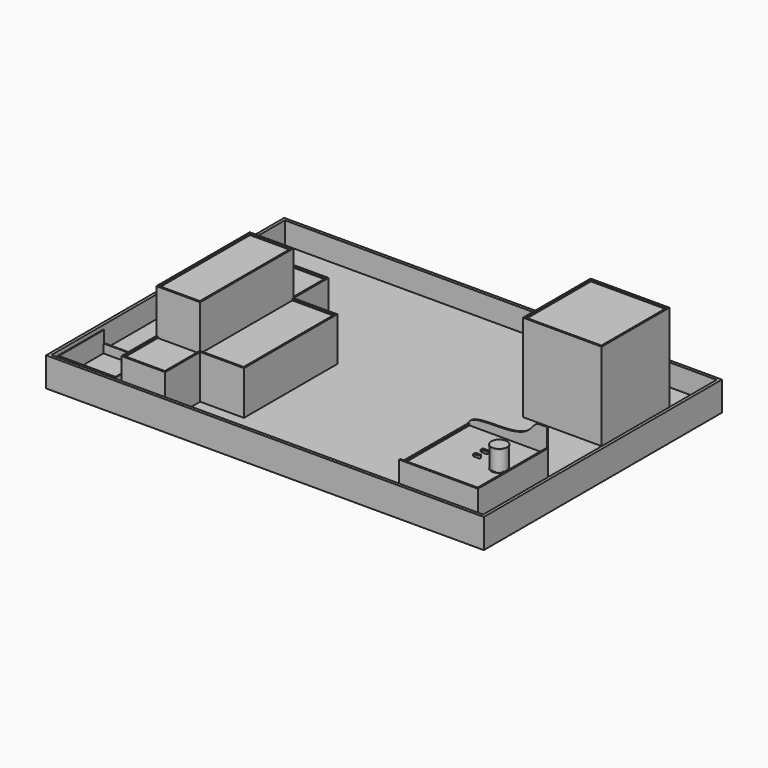
from build123d import *

# Parameters (mm, degrees)
F0_R      = 27.2
F1_DEPTH  = 2.83
F2_R      = 26.4
F3_DEPTH  = 67.36
F4_R      = 27.2
F5_DEPTH  = 2.83
F9_W      = 270
F9_H      = 300
F10_DEPTH = 72
F12_DEPTH = 15
F14_DEPTH = 5
F15_W     = 5
F15_H     = 290
F16_DEPTH = 5
F17_W     = 1500
F17_H     = 1020
F18_DEPTH = 25
F19_W     = 270
F19_H     = 290
F20_DEPTH = 300
F21_W     = 260
F21_H     = 280
F22_DEPTH = 5
F23_W     = 1500
F23_H     = 1020
F23_W_2   = 1480
F23_H_2   = 1000
F24_DEPTH = 75
F26_DEPTH = 150
F27_W     = 150
F27_H     = 400
F28_DEPTH = 150
F29_W     = 140
F29_H     = 390
F30_DEPTH = 5
F31_W     = 140
F31_H     = 145
F31_W_2   = 145
F31_H_2   = 390
F32_DEPTH = 5
F33_R     = 3
F34_DEPTH = 4
F35_R     = 3.99999
F35_2_R   = 3.99999
F36_R     = 3
F37_DEPTH = 8
F38_R     = 3
F39_DEPTH = 8
F40_R     = 3
F40_R_2   = 2.5
F41_DEPTH = 3
F42_R     = 3
F42_R_2   = 2.5
F43_DEPTH = 3
F45_DEPTH = 270.001
F46_W     = 200
F46_H     = 200
F46_W_2   = 194
F46_H_2   = 191
F47_DEPTH = 30
F49_DEPTH = 40
F50_R     = 2.5
F51_DEPTH = 8


# Not quite as in the source:
# - a fillet or chamfer is up to 0.001 mm smaller than in the source, because OpenCascade refuses the exact size
# - a feature names something its author has since deleted; it is built from what else it names


with BuildPart() as f1:
    # F0 (on Top) → F1 (new body)
    with BuildSketch(Plane.XY):
        Circle(F0_R)
    extrude(amount=F1_DEPTH)

    # F2 (on face) → F3 (join)
    with BuildSketch(Plane.XY.offset(2.83)):
        Circle(F2_R)
    extrude(amount=F3_DEPTH)

    # F4 (on face) → F5 (join)
    with BuildSketch(Plane.XY.offset(70.19)):
        Circle(F4_R)
    extrude(amount=F5_DEPTH)


with BuildPart() as f10:
    # F9 (on Top) → F10 (new body)
    with BuildSketch(Plane.XY):
        with Locations((-87.8, 0)):
            Rectangle(F9_W, F9_H)
    extrude(amount=-F10_DEPTH)

    # F11 (on face) → F12 (join)
    with BuildSketch(Plane.XY):
        Polygon((-222.8, -145), (-222.8, -150), (47.2, -150), (47.2, 150), (42.2, 150), (42.2, -145), align=None)
    extrude(amount=F12_DEPTH)

    # F13 (on face) → F14 (join)
    with BuildSketch(Plane(origin=(0, 150, 0), x_dir=(-1, 0, 0), z_dir=(0, 1, 0))):
        with BuildLine():
            Line((-21.3134280931, 81.3575685024), (-47.2, 81.3575685024))
            Line((-47.2, 81.3575685024), (-47.2, -72))
            Line((-47.2, -72), (222.8, -72))
            Line((222.8, -72), (222.8, 0))
            add(Edge.make_bspline(
                [(-21.3134280931, 81.3575685024), (-6.3059147253, 81.3822787863), (12.9585432644, 38.1268753575), (103.6097013063, 23.6068887567), (223.0224295336, 30.7718731823), (222.8, 0)],
                knots=[0, 0, 0, 0, 0.2487100673, 0.6151112321, 1, 1, 1, 1], degree=3))
        make_face()
    extrude(amount=-F14_DEPTH)

    # F15 (on face) → F16 (join)
    with BuildSketch(Plane.XY):
        with Locations((-220.3, 0)):
            Rectangle(F15_W, F15_H)
    extrude(amount=F16_DEPTH)

    # F17 (on face) → F18 (join)
    with BuildSketch(Plane(origin=(0, 0, -72), x_dir=(1, 0, 0), z_dir=(0, 0, -1))):
        with Locations((-602.8, -260)):
            Rectangle(F17_W, F17_H)
    extrude(amount=F18_DEPTH)

    # F19 (on face) → F20 (join)
    with BuildSketch(Plane.XY.offset(-72)):
        with Locations((-87.8, 525)):
            Rectangle(F19_W, F19_H)
    extrude(amount=F20_DEPTH)

    # F21 (on face) → F22 (cut)
    with BuildSketch(Plane.XY.offset(228)):
        with Locations((-87.8, 525)):
            Rectangle(F21_W, F21_H)
    extrude(amount=-F22_DEPTH, mode=Mode.SUBTRACT)

    # F23 (on face) → F24 (join)
    with BuildSketch(Plane.XY.offset(-72)):
        with Locations((-602.8, 260)):
            Rectangle(F23_W, F23_H)
        with Locations((-602.8, 260)):
            Rectangle(F23_W_2, F23_H_2, mode=Mode.SUBTRACT)
    extrude(amount=F24_DEPTH)

    # F25 (on face) → F26 (join)
    with BuildSketch(Plane.XY.offset(-72)):
        Polygon((-952.8, 460), (-1102.8, 460), (-1102.8, -240), (-952.8, -240), (-952.8, -90), (-802.8, -90), (-802.8, 310), (-952.8, 310), align=None)
    extrude(amount=F26_DEPTH)

    # F27 (on face) → F28 (join)
    with BuildSketch(Plane.XY.offset(78)):
        with Locations((-1027.8, 110)):
            Rectangle(F27_W, F27_H)
    extrude(amount=F28_DEPTH)

    # F29 (on face) → F30 (cut)
    with BuildSketch(Plane.XY.offset(228)):
        with Locations((-1027.8, 110)):
            Rectangle(F29_W, F29_H)
    extrude(amount=-F30_DEPTH, mode=Mode.SUBTRACT)

    # F31 (on face) → F32 (cut)
    with BuildSketch(Plane.XY.offset(78)):
        with Locations((-1027.8, 382.5)):
            Rectangle(F31_W, F31_H)
        with Locations((-880.3, 110)):
            Rectangle(F31_W_2, F31_H_2)
        with Locations((-1027.8, -162.5)):
            Rectangle(F31_W, F31_H)
    extrude(amount=-F32_DEPTH, mode=Mode.SUBTRACT)

    # F46 (on face) → F47 (join)
    with BuildSketch(Plane.XY.offset(-72)):
        with Locations((-1232.8, -130)):
            Rectangle(F46_W, F46_H)
        with Locations((-1232.8, -128.5)):
            Rectangle(F46_W_2, F46_H_2, mode=Mode.SUBTRACT)
    extrude(amount=F47_DEPTH)

    # F48 (on face) → F49 (join)
    with BuildSketch(Plane.XY.offset(-42)):
        Polygon((-1329.8, -30), (-1332.8, -30), (-1332.8, -230), (-1329.8, -230), (-1135.8, -230), (-1132.8, -230), (-1132.8, -30), (-1135.8, -30), (-1135.8, -224), (-1329.8, -224), align=None)
    extrude(amount=F49_DEPTH)


with BuildPart() as f34:
    # F33 (on offset) → F34 (new body, symmetric)
    with BuildSketch(Plane.XY.offset(25)):
        with BuildLine():
            Line((-55, -12), (-74.5, -12))
            Line((-74.5, -12), (-74.5, -13))
            Line((-74.5, -13), (-65.6457513111, -13))
            ThreePointArc((-65.6457513111, -13), (-67, -16), (-65.6457513111, -19))
            Line((-65.6457513111, -19), (-74.5, -19))
            Line((-74.5, -19), (-74.5, -20))
            Line((-74.5, -20), (-55, -20))
            ThreePointArc((-55, -20), (-51, -16), (-55, -12))
        make_face()
        with Locations((-63, -16)):
            Circle(F33_R, mode=Mode.SUBTRACT)
        with Locations((-55, -16)):
            Circle(F33_R, mode=Mode.SUBTRACT)
    extrude(amount=F34_DEPTH, both=True)

    # F35 (radius 4 in the source; OpenCascade refuses exactly that, so slightly less here)
    f35_edges = [f34.edges().sort_by_distance(p)[0] for p in [
        (-74.5, -19.5, 29),
        (-74.5, -12.5, 29),
        (-74.5, -19.5, 21),
        (-74.5, -12.5, 21),
    ]]
    fillet(f35_edges, radius=F35_R)

    # F36 (on face) → F37 (join, through all)
    with BuildSketch(Plane.XZ.offset(20)):
        with Locations((-70.5, 25)):
            Circle(F36_R)
    extrude(amount=-F37_DEPTH)

    # F42 (on offset) → F43 (join, symmetric)
    with BuildSketch(Plane.XY.offset(25)):
        with Locations((-63, -16)):
            Circle(F42_R)
        with Locations((-63, -16)):
            Circle(F42_R_2, mode=Mode.SUBTRACT)
        with Locations((-55, -16)):
            Circle(F42_R)
        with Locations((-55, -16)):
            Circle(F42_R_2, mode=Mode.SUBTRACT)
    extrude(amount=F43_DEPTH, both=True)


with BuildPart() as f34b:
    # F33 (on offset) → F34, piece 2 (new body, symmetric)
    with BuildSketch(Plane.XY.offset(25)):
        with BuildLine():
            Line((-74.5, 13), (-74.5, 12))
            Line((-74.5, 12), (-55, 12))
            ThreePointArc((-55, 12), (-51, 16), (-55, 20))
            Line((-55, 20), (-74.5, 20))
            Line((-74.5, 20), (-74.5, 19))
            Line((-74.5, 19), (-65.6457513111, 19))
            ThreePointArc((-65.6457513111, 19), (-67, 16), (-65.6457513111, 13))
            Line((-65.6457513111, 13), (-74.5, 13))
        make_face()
        with Locations((-63, 16)):
            Circle(F33_R, mode=Mode.SUBTRACT)
        with Locations((-55, 16)):
            Circle(F33_R, mode=Mode.SUBTRACT)
    extrude(amount=F34_DEPTH, both=True)

    # F35#2 (radius 4 in the source; OpenCascade refuses exactly that, so slightly less here)
    f35_2_edges = [f34b.edges().sort_by_distance(p)[0] for p in [
        (-74.5, 12.5, 29),
        (-74.5, 19.5, 29),
        (-74.5, 19.5, 21),
        (-74.5, 12.5, 21),
    ]]
    fillet(f35_2_edges, radius=F35_2_R)

    # F38 (on face) → F39 (join, through all)
    with BuildSketch(Plane(origin=(0, 20, 0), x_dir=(-1, 0, 0), z_dir=(0, 1, 0))):
        with Locations((70.5, 25)):
            Circle(F38_R)
    extrude(amount=-F39_DEPTH)

    # F40 (on offset) → F41 (join, symmetric)
    with BuildSketch(Plane.XY.offset(25)):
        with Locations((-55, 16)):
            Circle(F40_R)
        with Locations((-55, 16)):
            Circle(F40_R_2, mode=Mode.SUBTRACT)
        with Locations((-63, 16)):
            Circle(F40_R)
        with Locations((-63, 16)):
            Circle(F40_R_2, mode=Mode.SUBTRACT)
    extrude(amount=F41_DEPTH, both=True)


with BuildPart() as f45_tool:
    # F44 (on face) → F45 (new body, through all)
    with BuildSketch(Plane(origin=(0, 20, 0), x_dir=(-1, 0, 0), z_dir=(0, 1, 0))):
        with BuildLine():
            Line((71.5, 26), (71.5, 27.2912878475))
            ThreePointArc((71.5, 27.2912878475), (70.5, 27.5), (69.5, 27.2912878475))
            Line((69.5, 27.2912878475), (69.5, 26))
            Line((69.5, 26), (68.2087121525, 26))
            ThreePointArc((68.2087121525, 26), (68, 25), (68.2087121525, 24))
            Line((68.2087121525, 24), (69.5, 24))
            Line((69.5, 24), (69.5, 22.7087121525))
            ThreePointArc((69.5, 22.7087121525), (70.5, 22.5), (71.5, 22.7087121525))
            Line((71.5, 22.7087121525), (71.5, 24))
            Line((71.5, 24), (72.7912878475, 24))
            ThreePointArc((72.7912878475, 24), (73, 25), (72.7912878475, 26))
            Line((72.7912878475, 26), (71.5, 26))
        make_face()
    extrude(amount=-F45_DEPTH)


with BuildPart() as f34_1:
    add(f34.part)

    # F45: cut by f45_tool
    add(f45_tool.part, mode=Mode.SUBTRACT)


with BuildPart() as f34b_1:
    add(f34b.part)

    # F45: cut by f45_tool
    add(f45_tool.part, mode=Mode.SUBTRACT)


with BuildPart() as f51:
    # F50 (on face) → F51 (new body)
    with BuildSketch(Plane.XY.offset(29)):
        Polygon((-0.619225204, 27.0833074003), (-78.9677798748, 27.0833074003), (-78.9677798748, 12), (-44.8230803013, 12), (-44.8230803013, -8.2436139807), (-78.9677798748, -8.2436139807), (-78.9677798748, -29.8999884278), (-0.619225204, -29.8999884278), align=None)
        with Locations((-63, 16)):
            Circle(F50_R, mode=Mode.SUBTRACT)
    extrude(amount=F51_DEPTH)


solid = Compound([f1.part, f10.part, f34_1.part, f34b_1.part])
